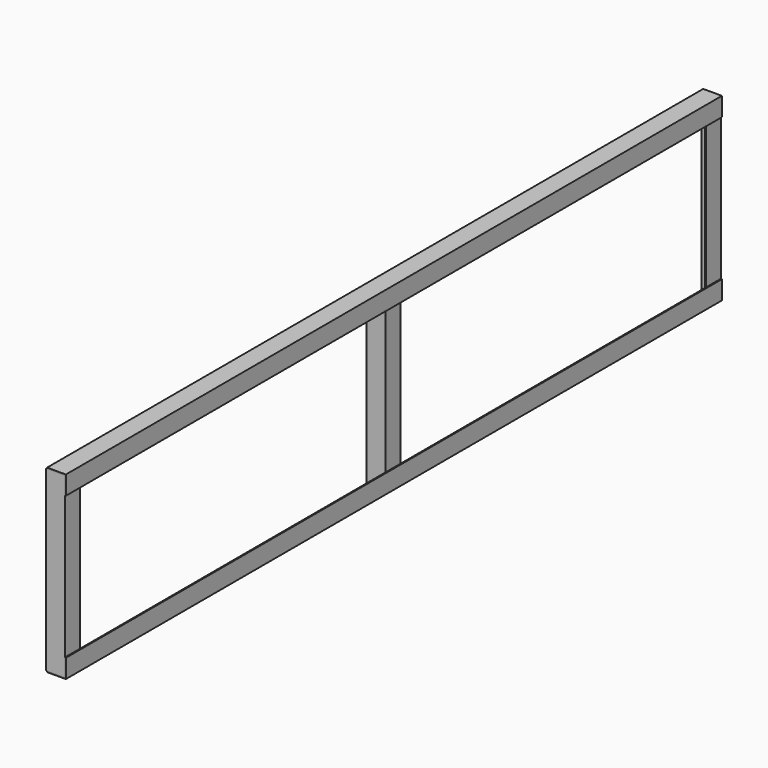
from build123d import *

# Parameters (mm, degrees)
F1_DEPTH = 2222.5
F3_DEPTH = 482.6


# Not quite as in the source:
# - a feature of the source that left no trace in its solid (it failed there, or was rolled back) is left out
# - a pattern or mirror of a feature is missing from the dataset's text; its kind, count and spacing are read off the source's solid


with BuildPart() as f1:
    # F0 (on Front) → F1 (new body)
    with BuildSketch(Plane.XZ):
        Polygon((-50.8, 0), (0, 0), (0, 50.8), (-2.7686, 50.8), (-2.7686, 2.7686), (-50.8, 2.7686), align=None)
    extrude(amount=-F1_DEPTH)


with BuildPart() as f3:
    # F2 (on face) → F3 (new body)
    with BuildSketch(Plane.XY.offset(2.7686)):
        Polygon((-2.7686, 2171.7), (-2.7686, 2222.5), (-53.5686, 2222.5), (-53.5686, 2219.7314), (-5.5372, 2219.7314), (-5.5372, 2171.7), align=None)
    extrude(amount=F3_DEPTH)


with BuildPart() as f3_copies_1:
    # F3_copies: instance of F3
    add(f3.part.mirror(Plane(origin=(0, 1654.175, 0), x_dir=(0, 0, -1), z_dir=(0, -1, 0))))


with BuildPart() as f5_1:
    # F5: instance of F3
    add(f3.part.mirror(Plane.XZ.offset(-1111.25)))


with BuildPart() as f7_1:
    # F7: instance of F1
    add(f1.part.mirror(Plane.XY.offset(244.0686)))


solid = Compound([f1.part, f3.part, f3_copies_1.part, f5_1.part, f7_1.part])
